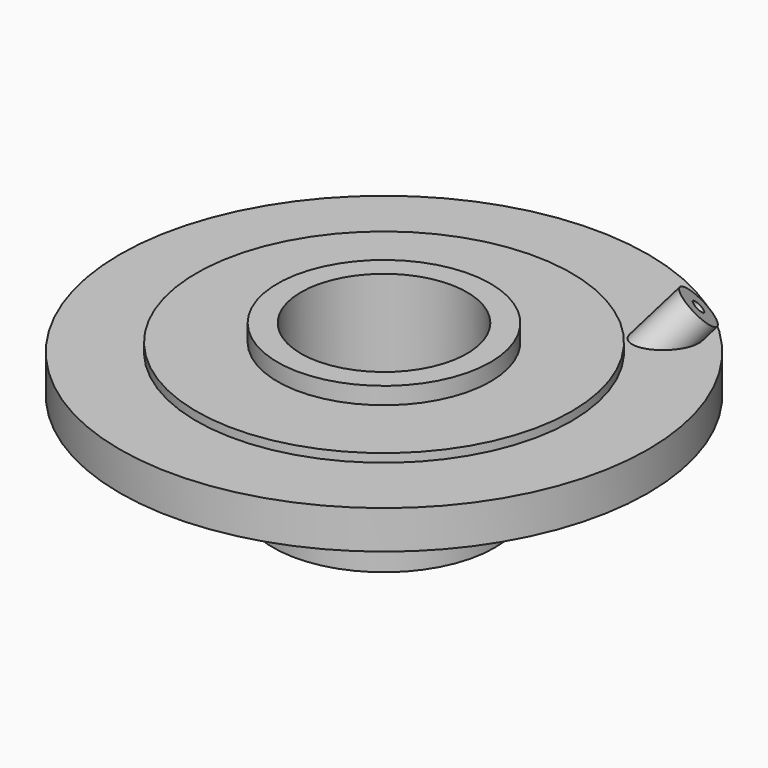
from build123d import *

# Parameters (mm, degrees)
F0_W      = 635
F0_H      = 101.6
F0_W_2    = 660.4
F0_H_2    = 508
F3_D      = 990.6
F9_R      = 38.1
F10_REACH = 3406.7732486981


# Not quite as in the source:
# - a feature names something its author has since deleted; it is built from what else it names


with BuildPart() as f1:
    # F0 (on Front) → F1 (revolve)
    with BuildSketch(Plane.XZ):
        with Locations((317.5, 50.8)):
            Rectangle(F0_W, F0_H)
        Polygon((635, 0), (0, 0), (0, -50.8), (1117.6, -50.8), (1117.6, 0), align=None)
        Polygon((1117.6, -50.8), (0, -50.8), (0, -279.4), (774.7, -279.4), (1574.8, -279.4), (1574.8, -50.8), align=None)
        Polygon((774.7, -279.4), (0, -279.4), (0, -355.6), (660.4, -355.6), (774.7, -355.6), align=None)
        with Locations((330.2, -609.6)):
            Rectangle(F0_W_2, F0_H_2)
    revolve(axis=Axis((0, 0, -260.6765925884), (0, 0, -1)))

    # F3 (through all)
    with Locations(Plane.XY.offset(101.6)):
        with Locations((0, 0)):
            Hole(F3_D / 2)

    # F6 (on face) → F7 (revolve)
    with BuildSketch(Plane(origin=(0, 0, 0), x_dir=(0.7071067812, 0.7071067812, 0), z_dir=(0.7071067812, -0.7071067812, 0))):
        Polygon((1321.5041428375, -50.0958571625), (1473.2, 101.6), (1383.3974387893, 191.4025612107), (1141.8990204161, -50.0958571625), align=None)
    revolve(axis=Axis((867.2468509569, 867.2468509569, -145.1277414514), (-0.5, -0.5, -0.7071067812)))

    f10_end = Plane(origin=(-16.75319514, -16.75319514, -50.8), x_dir=(1, 0, 0), z_dir=(0, 0, 1))
    # F9 (on face) → F10 (cut, up to a plane its end follows)
    with BuildSketch(Plane(origin=(556.7758795063, 556.7758795063, 787.4), x_dir=(0.8660254038, -0.2886751346, -0.4082482905), z_dir=(0.5, 0.5, 0.7071067812))):
        with Locations((559.9533552002, 791.8936292205)):
            Circle(F9_R)
    f10_long = extrude(amount=-F10_REACH, mode=Mode.PRIVATE)
    add(split(f10_long, bisect_by=f10_end, keep=Keep.TOP, mode=Mode.PRIVATE), mode=Mode.SUBTRACT)


solid = f1.part
